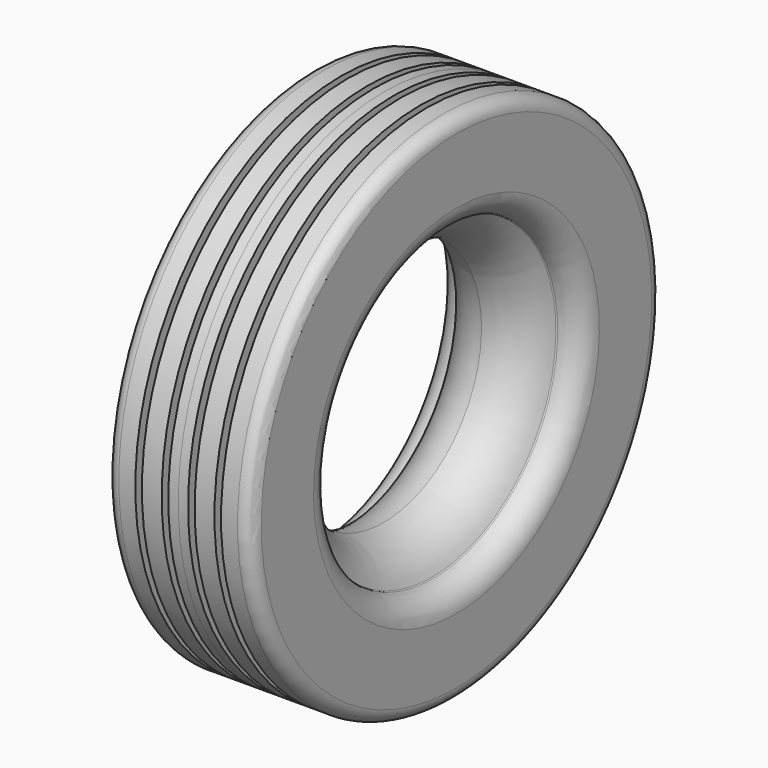
from build123d import *
from build123d import SkipClean  # not in build123d's __all__


with BuildPart() as f1:
    # F0 (on Front) → F1 (revolve)
    with BuildSketch(Plane.XZ):
        with BuildLine():
            Line((25, 390), (25, 375))
            Line((25, 375), (15, 375))
            Line((15, 375), (15, 390))
            Line((15, 390), (0, 390))
            Line((0, 390), (0, 185))
            ThreePointArc((0, 185), (44.1831956873, 198.3078324025), (73.6668272943, 233.8038695285))
            ThreePointArc((73.6668272943, 233.8038695285), (74.3744217546, 234.6713493802), (75.4373254745, 235.0226994843))
            ThreePointArc((75.4373254745, 235.0226994843), (99.9502477461, 245.9516970753), (110, 270.838015129))
            Line((110, 270.838015129), (110, 370))
            ThreePointArc((110, 370), (104.1421356237, 384.1421356237), (90, 390))
            Line((90, 390), (65, 390))
            Line((65, 390), (65, 375))
            Line((65, 375), (55, 375))
            Line((55, 375), (55, 390))
            Line((55, 390), (25, 390))
        make_face()
    revolve(axis=Axis((33.0590110619, 0, 0), (1, 0, 0)))

    # F2: F1 across face


with BuildPart() as f1_1:
    add(f1.part, clean=False)
    with SkipClean():  # cleaning this boolean's faces spoils the solid; the shape is the same uncleaned
        add(f1.part.mirror(Plane(origin=(0, 0, 0), x_dir=(0, -1, 0), z_dir=(-1, 0, 0))), clean=False)


solid = f1_1.part
